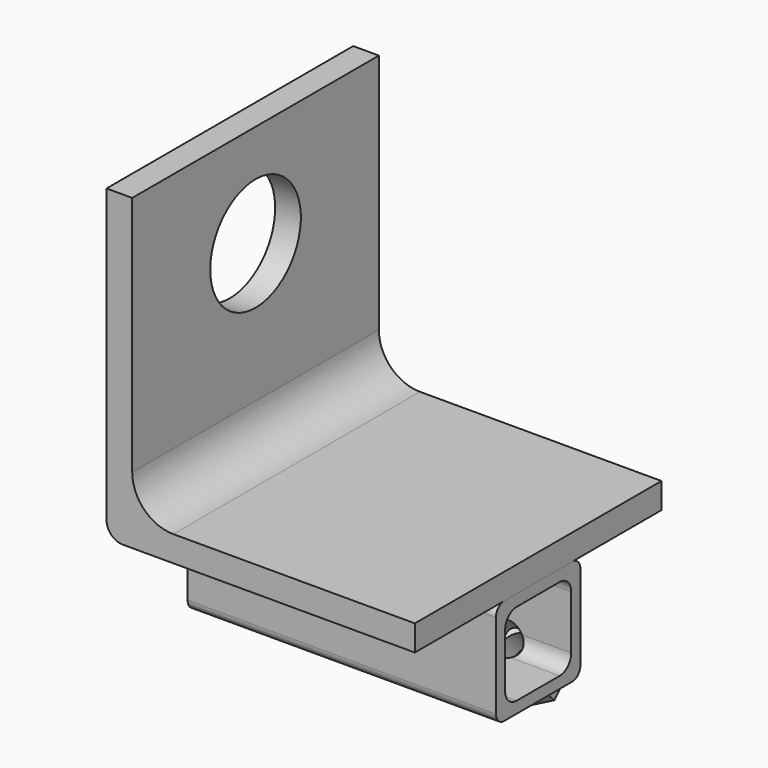
from build123d import *

# Parameters (mm, degrees)
F1_DEPTH  = 38.1
F2_R      = 6.9977
F3_DEPTH  = 38.101
F4_R      = 2.032
F5_R      = 5.08
F6_W      = 13.0556
F6_H      = 13.0556
F7_DEPTH  = 38.1
F8_T      = -1.4224
F9_R      = 1.27
F10_R     = 1.778
F12_R     = 1.984375
F13_DEPTH = 17.1892102157
F16_R     = 1.984375
F17_DEPTH = 3.302
F18_R     = 0.254
F18_2_R   = 0.254


with BuildPart() as f1:
    # F0 (on Front) → F1 (new body)
    with BuildSketch(Plane.XZ):
        Polygon((3.175, 38.1), (0, 38.1), (0, 0), (38.1, 0), (38.1, 3.175), (3.175, 3.175), align=None)
    extrude(amount=F1_DEPTH)

    # F2 (on face) → F3 (cut, through all)
    with BuildSketch(Plane(origin=(0, 0, 0), x_dir=(0, -1, 0), z_dir=(-1, 0, 0))):
        with Locations((19.05, 25.4)):
            Circle(F2_R)
    extrude(amount=-F3_DEPTH, mode=Mode.SUBTRACT)

    # F4
    f4_edges = [f1.edges().sort_by_distance(p)[0] for p in [
        (0, -19.05, 0),
    ]]
    fillet(f4_edges, radius=F4_R)

    # F5
    f5_edges = [f1.edges().sort_by_distance(p)[0] for p in [
        (3.175, -19.05, 3.175),
    ]]
    fillet(f5_edges, radius=F5_R)


with BuildPart() as f7:
    # F6 (on face) → F7 (new body, through all)
    with BuildSketch(Plane(origin=(0, 0, 0), x_dir=(0, -1, 0), z_dir=(-1, 0, 0))):
        with Locations((19.05, -6.5278)):
            Rectangle(F6_W, F6_H)
    extrude(amount=-F7_DEPTH)

    # F8
    f8_openings = [f7.faces().sort_by_distance(p)[0] for p in [
        (38.1, -19.05, -6.5278),
        (0, -19.05, -6.5278),
    ]]
    offset(amount=F8_T, openings=f8_openings)

    # F9
    f9_edges = [f7.edges().sort_by_distance(p)[0] for p in [
        (19.05, -25.5778, -13.0556),
        (19.05, -25.5778, 0),
        (19.05, -12.5222, -13.0556),
        (19.05, -12.5222, 0),
    ]]
    fillet(f9_edges, radius=F9_R)

    # F10
    f10_edges = [f7.edges().sort_by_distance(p)[0] for p in [
        (19.05, -24.1554, -11.6332),
        (19.05, -24.1554, -1.4224),
        (19.05, -13.9446, -1.4224),
        (19.05, -13.9446, -11.6332),
    ]]
    fillet(f10_edges, radius=F10_R)

    # F12 (on face) → F13 (cut, through all)
    with BuildSketch(Plane(origin=(0, -5.6261, 5.6261), x_dir=(1, 0, 0), z_dir=(0, -0.7071067812, 0.7071067812))):
        with Locations((30.48, -18.0862358278)):
            Circle(F12_R)
        with Locations((7.62, -18.0862358278)):
            Circle(F12_R)
    extrude(amount=-F13_DEPTH, mode=Mode.SUBTRACT)


with BuildPart() as f17:
    # F16 (on face) → F17 (new body)
    with BuildSketch(Plane(origin=(0, -0.1052743879, 0.1052743879), x_dir=(1, 0, 0), z_dir=(0, -0.7071067812, 0.7071067812))):
        Polygon((11.985625, -20.6067305968), (11.985625, -15.5657410589), (7.62, -13.04524629), (3.254375, -15.5657410589), (3.254375, -20.6067305968), (7.62, -23.1272253657), align=None)
        with Locations((7.62, -18.0862358278)):
            Circle(F16_R, mode=Mode.SUBTRACT)
    extrude(amount=-F17_DEPTH)

    # F18
    f18_edges = [f17.edges().sort_by_distance(p)[0] for p in [
        (9.802812, -13.232696, -17.691881),
        (11.985625, -10.559308, -15.018492),
        (9.802812, -7.885919, -12.345104),
        (5.437187, -7.885919, -12.345104),
        (3.254375, -10.559308, -15.018492),
        (5.437188, -13.232696, -17.691881),
        (5.635625, -10.559308, -15.018492),
    ]]
    fillet(f18_edges, radius=F18_R)


with BuildPart() as f17b:
    # F16 (on face) → F17, piece 2 (new body)
    with BuildSketch(Plane(origin=(0, -0.1052743879, 0.1052743879), x_dir=(1, 0, 0), z_dir=(0, -0.7071067812, 0.7071067812))):
        Polygon((34.845625, -15.5657410589), (30.48, -13.04524629), (26.114375, -15.5657410589), (26.114375, -20.6067305968), (30.48, -23.1272253657), (34.845625, -20.6067305968), align=None)
        with Locations((30.48, -18.0862358278)):
            Circle(F16_R, mode=Mode.SUBTRACT)
    extrude(amount=-F17_DEPTH)

    # F18#2
    f18_2_edges = [f17b.edges().sort_by_distance(p)[0] for p in [
        (34.845625, -10.559308, -15.018492),
        (32.662813, -7.885919, -12.345104),
        (28.297187, -7.885919, -12.345104),
        (26.114375, -10.559308, -15.018492),
        (28.297187, -13.232696, -17.691881),
        (32.662813, -13.232696, -17.691881),
        (28.495625, -10.559308, -15.018492),
    ]]
    fillet(f18_2_edges, radius=F18_2_R)


solid = Compound([f1.part, f7.part, f17.part, f17b.part])
